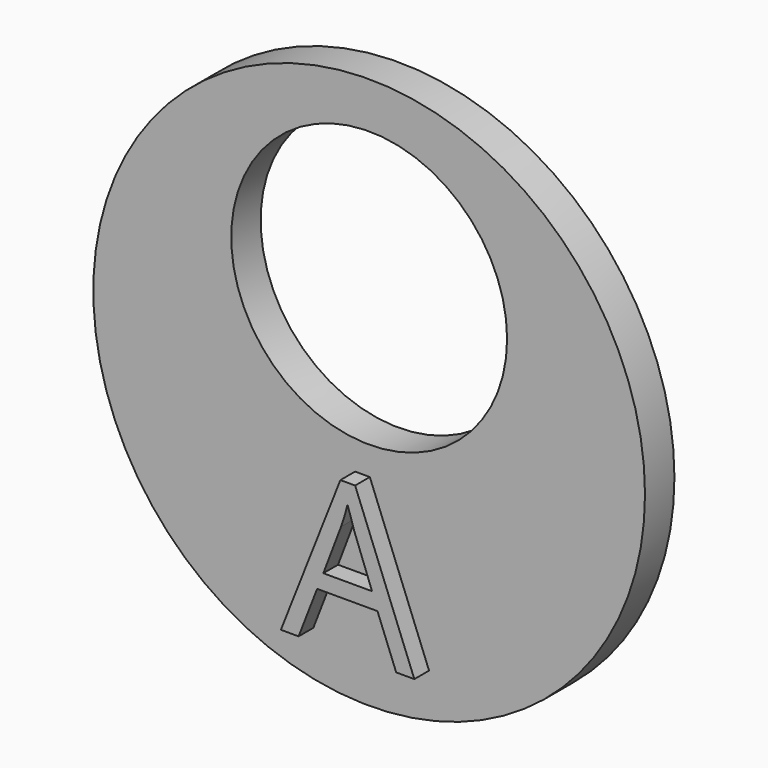
from build123d import *

# Parameters (mm, degrees)
F0_R         = 15
F0_R_2       = 7.5
F1_DEPTH     = 2
F2_TEXT_SIZE = 11.4669652856
F3_DEPTH     = 1


# Not quite as in the source:
# - Text() gives the source's letters only with a copy of the font that has no kerning and outlines rounded to 1/6400 em; it was checked with that copy


with BuildPart() as f1:
    # F0 (on Front) → F1 (new body)
    with BuildSketch(Plane.XZ):
        Circle(F0_R)
        with Locations((0, 5)):
            Circle(F0_R_2, mode=Mode.SUBTRACT)
    extrude(amount=F1_DEPTH)

    # F2 (on face) → F3 (join)
    with BuildSketch(Plane.XZ.offset(2)):
        with Locations((-4, -12.2562150056)):
            Text('A', F2_TEXT_SIZE, font='Open Sans', text_align=(TextAlign.LEFT, TextAlign.BOTTOM))
    extrude(amount=F3_DEPTH)


solid = f1.part
